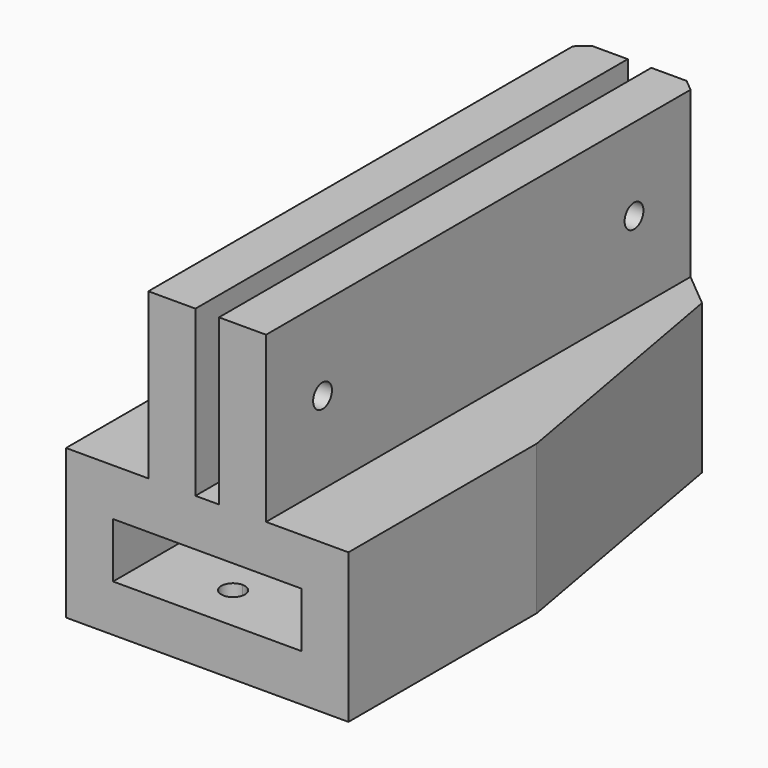
from build123d import *

# Parameters (mm, degrees)
F0_W     = 2
F0_H     = 10
F1_DEPTH = 2.3368
F2_DEPTH = 2.0066
F4_DEPTH = 2
F6_DEPTH = 7
F8_D     = 1


# Not quite as in the source:
# - a feature names something its author has since deleted; it is built from what else it names


with BuildPart() as f1:
    # F0 (on Top) → F1 (new body)
    with BuildSketch(Plane.XY):
        with Locations((-18.8875418854, 5)):
            Rectangle(F0_W, F0_H)
        with Locations((-8.8875418854, 5)):
            Rectangle(F0_W, F0_H)
        Polygon((-17.8550429996, 21.3176092022), (-15.8875418854, 20.9585279226), (-15.8875418854, 22.9585279226), align=None)
        Polygon((-11.8875418854, 22.9585279226), (-11.8875418854, 20.9585279226), (-9.9200407711, 21.3176092022), align=None)
        Polygon((-11.8875418854, 20.9585279226), (-9.8875418854, 10), (-7.8875418854, 10), (-9.9200407711, 21.3176092022), align=None)
        Polygon((-15.8875418854, 20.9585279226), (-13.8875418854, 20.9585279226), (-11.8875418854, 20.9585279226), (-11.8875418854, 22.9585279226), (-15.8875418854, 22.9585279226), align=None)
        Polygon((-19.8875418854, 10), (-17.8875418854, 10), (-15.8875418854, 20.9585279226), (-17.8550429996, 21.3176092022), align=None)
    extrude(amount=-F1_DEPTH)

    # F0 (on Top) → F2 (join)
    with BuildSketch(Plane.XY):
        Polygon((-17.8875418854, 10), (-17.8875418854, 0), (-13.8875418854, 0), (-13.8875418854, 20.9585279226), (-15.8875418854, 20.9585279226), align=None)
        with Locations((-18.8875418854, 5)):
            Rectangle(F0_W, F0_H)
        Polygon((-13.8875418854, 20.9585279226), (-13.8875418854, 0), (-9.8875418854, 0), (-9.8875418854, 10), (-11.8875418854, 20.9585279226), align=None)
        Polygon((-19.8875418854, 10), (-17.8875418854, 10), (-15.8875418854, 20.9585279226), (-17.8550429996, 21.3176092022), align=None)
        with Locations((-8.8875418854, 5)):
            Rectangle(F0_W, F0_H)
        Polygon((-15.8875418854, 20.9585279226), (-13.8875418854, 20.9585279226), (-11.8875418854, 20.9585279226), (-11.8875418854, 22.9585279226), (-15.8875418854, 22.9585279226), align=None)
        Polygon((-17.8550429996, 21.3176092022), (-15.8875418854, 20.9585279226), (-15.8875418854, 22.9585279226), align=None)
        Polygon((-11.8875418854, 20.9585279226), (-9.8875418854, 10), (-7.8875418854, 10), (-9.9200407711, 21.3176092022), align=None)
        Polygon((-11.8875418854, 22.9585279226), (-11.8875418854, 20.9585279226), (-9.9200407711, 21.3176092022), align=None)
    extrude(amount=F2_DEPTH)

    # F3 (on face) → F4 (join)
    with BuildSketch(Plane(origin=(0, 0, -2.3368), x_dir=(1, 0, 0), z_dir=(0, 0, -1))):
        Polygon((-14.3875418854, 0), (-17.8875418854, 0), (-17.8875418854, -10), (-15.8875418854, -20.9585279226), (-11.8875418854, -20.9585279226), (-9.8875418854, -10), (-9.8875418854, 0), align=None)
        with BuildLine():
            ThreePointArc((-13.8875418854, -11), (-14.7410952759, -11.3535533906), (-14.3875418854, -10.5))
            ThreePointArc((-14.3875418854, -10.5), (-14.0339884948, -10.6464466094), (-13.8875418854, -11))
        make_face(mode=Mode.SUBTRACT)
        with BuildLine():
            ThreePointArc((-14.3875418854, -2.5), (-14.8875418854, -2), (-14.3875418854, -1.5))
            ThreePointArc((-14.3875418854, -1.5), (-14.0339884948, -1.6464466094), (-13.8875418854, -2))
            ThreePointArc((-13.8875418854, -2), (-14.0339884948, -2.3535533906), (-14.3875418854, -2.5))
        make_face(mode=Mode.SUBTRACT)
        Polygon((-17.8875418854, 0), (-19.8875418854, 0), (-19.8875418854, -10), (-17.8550429996, -21.3176092022), (-15.8875418854, -22.9585279226), (-11.8875418854, -22.9585279226), (-9.9200407711, -21.3176092022), (-7.8875418854, -10), (-7.8875418854, 0), (-9.8875418854, 0), (-9.8875418854, -10), (-11.8875418854, -20.9585279226), (-15.8875418854, -20.9585279226), (-17.8875418854, -10), align=None)
    extrude(amount=F4_DEPTH)

    # F5 (on face) → F6 (join)
    with BuildSketch(Plane.XY.offset(2.0066)):
        Polygon((-13.3875418854, 22.9585279226), (-13.3875418854, 0), (-11.3875418854, 0), (-11.3875418854, 22.5415221307), (-11.8875418854, 22.9585279226), align=None)
        Polygon((-16.3875418854, 0), (-14.3875418854, 0), (-14.3875418854, 22.9585279226), (-15.8875418854, 22.9585279226), (-16.3875418854, 22.5415221307), align=None)
    extrude(amount=F6_DEPTH)

    # F8 (through all)
    with Locations(Plane.YZ.offset(-11.3875418854)):
        with Locations((3, 5.5066), (19.5415221307, 5.5066)):
            Hole(F8_D / 2)


solid = f1.part
